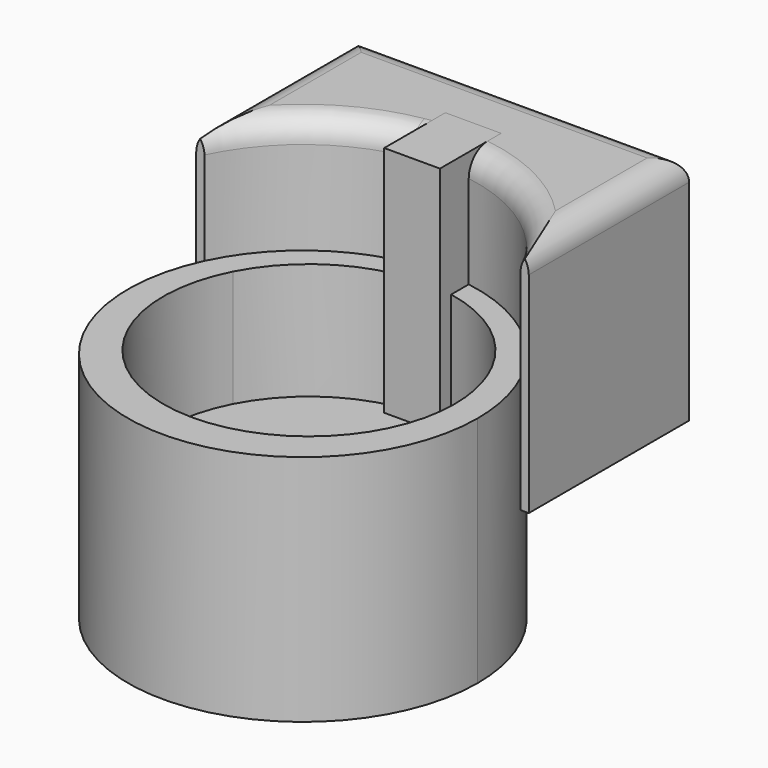
from build123d import *

# Parameters (mm, degrees)
F1_DEPTH    = 50.8
F2_DEPTH    = 25.4
F3_DEPTH    = 25.4
F4_T1_DEPTH = 97.86927917
F4_T3_DEPTH = 69.072270802
F4_T6_ANGLE = 93.763795783
F4_T8_ANGLE = 93.763795783
F5_DEPTH    = 50.8


# Not quite as in the source:
# - a fillet or chamfer that OpenCascade refuses, or shapes differently, is made with other operations: its cross-section is extruded or revolved along the edge and cut away or added


with BuildPart() as f1:
    # F0 (on Top) → F1 (new body)
    with BuildSketch(Plane.XY):
        with BuildLine():
            ThreePointArc((6.0717510059, 35.9461629091), (22.9027694367, 28.7809581965), (34.4542698124, 14.5969468084))
            Line((34.4542698124, 14.5969468084), (36.234639585, 14.5969468084))
            Line((36.234639585, 14.5969468084), (36.234639585, 58.2692176104))
            Line((36.234639585, 58.2692176104), (-36.234639585, 58.2692176104))
            Line((-36.234639585, 58.2692176104), (-36.234639585, 14.5969468084))
            Line((-36.234639585, 14.5969468084), (-34.4542698124, 14.5969468084))
            ThreePointArc((-34.4542698124, 14.5969468084), (-22.9027694367, 28.7809581965), (-6.0717510059, 35.9461629091))
            Line((-6.0717510059, 35.9461629091), (-6.0717510059, 44.7598363188))
            Line((-6.0717510059, 44.7598363188), (6.0717510059, 44.7598363188))
            Line((6.0717510059, 44.7598363188), (6.0717510059, 35.9461629091))
        make_face()
    extrude(amount=F1_DEPTH)

    # F4: fillet of radius 5.08 on 5 edges, made by hand

    # F4_s2 → F4_t1 (cut)
    with BuildSketch(Plane.YZ.offset(-48.934639585)):
        with BuildLine():
            ThreePointArc((58.2692176104, 45.72), (56.7813200588, 49.3121024484), (53.1892176104, 50.8))
            Line((53.1892176104, 50.8), (58.2692176104, 50.8))
            Line((58.2692176104, 50.8), (58.2692176104, 45.72))
        make_face()
    extrude(amount=F4_T1_DEPTH, mode=Mode.SUBTRACT)

    # F4_s4 → F4_t3 (cut)
    with BuildSketch(Plane.XZ.offset(-70.9692176104)):
        with BuildLine():
            ThreePointArc((36.234639585, 45.72), (34.7467420334, 49.3121024484), (31.154639585, 50.8))
            Line((31.154639585, 50.8), (36.234639585, 50.8))
            Line((36.234639585, 50.8), (36.234639585, 45.72))
        make_face()
        with BuildLine():
            ThreePointArc((-36.234639585, 45.72), (-34.7467420334, 49.3121024484), (-31.154639585, 50.8))
            Line((-31.154639585, 50.8), (-36.234639585, 50.8))
            Line((-36.234639585, 50.8), (-36.234639585, 45.72))
        make_face()
    extrude(amount=F4_T3_DEPTH, mode=Mode.SUBTRACT)

    # F4_s5 → F4_t6 (revolve, cut)
    with BuildSketch(Plane(origin=(-0.2831878776, -0.0495849538, 0), x_dir=(0, 0, 1), z_dir=(-0.9850144718, -0.1724717085, 0))):
        with BuildLine():
            ThreePointArc((45.72, 36.4580618529), (49.3121024484, 37.9459594044), (50.8, 41.5380618529))
            Line((50.8, 41.5380618529), (50.8, 36.4580618529))
            Line((50.8, 36.4580618529), (45.72, 36.4580618529))
        make_face()
    revolve(axis=Axis((0, -1.6669177906, 50.8), (0, 0, -1)), revolution_arc=F4_T6_ANGLE, mode=Mode.SUBTRACT)

    # F4_s7 → F4_t8 (revolve, cut)
    with BuildSketch(Plane(origin=(-0.1780570086, -1.6476759621, 0), x_dir=(0, 0, 1), z_dir=(-0.1074400196, -0.9942115681, 0))):
        with BuildLine():
            ThreePointArc((45.72, 37.9209063199), (49.3121024484, 39.4088038715), (50.8, 43.0009063199))
            Line((50.8, 43.0009063199), (50.8, 37.9209063199))
            Line((50.8, 37.9209063199), (45.72, 37.9209063199))
        make_face()
    revolve(axis=Axis((0, -1.6669177906, 50.8), (0, 0, -1)), revolution_arc=F4_T8_ANGLE, mode=Mode.SUBTRACT)


with BuildPart() as f2:
    # F0 (on Top) → F2 (new body, symmetric)
    with BuildSketch(Plane.XY):
        with BuildLine():
            ThreePointArc((-34.4542698124, 14.5969468084), (-8.3337362614, -38.8443146861), (38.1, -1.6669177906))
            ThreePointArc((38.1, -1.6669177906), (37.1773968955, 6.6668184707), (34.4542698124, 14.5969468084))
            Line((34.4542698124, 14.5969468084), (28.1955961787, 14.5969468084))
            ThreePointArc((28.1955961787, 14.5969468084), (30.8486035233, 7.5117348637), (31.75, 0))
            ThreePointArc((31.75, 0), (-7.5117348637, -30.8486035233), (-28.1955961787, 14.5969468084))
            Line((-28.1955961787, 14.5969468084), (-34.4542698124, 14.5969468084))
        make_face()
        with BuildLine():
            Line((28.1955961787, 14.5969468084), (34.4542698124, 14.5969468084))
            ThreePointArc((34.4542698124, 14.5969468084), (22.9027694367, 28.7809581965), (6.0717510059, 35.9461629091))
            Line((6.0717510059, 35.9461629091), (6.0717510059, 31.1640231633))
            ThreePointArc((6.0717510059, 31.1640231633), (19.0310213994, 25.414222878), (28.1955961787, 14.5969468084))
        make_face()
        with BuildLine():
            ThreePointArc((-6.0717510059, 35.9461629091), (-22.9027694367, 28.7809581965), (-34.4542698124, 14.5969468084))
            Line((-34.4542698124, 14.5969468084), (-28.1955961787, 14.5969468084))
            ThreePointArc((-28.1955961787, 14.5969468084), (-19.0310213994, 25.414222878), (-6.0717510059, 31.1640231633))
            Line((-6.0717510059, 31.1640231633), (-6.0717510059, 35.9461629091))
        make_face()
    extrude(amount=F2_DEPTH, both=True)


with BuildPart() as f3:
    # F0 (on Top) → F3 (new body)
    with BuildSketch(Plane.XY):
        with BuildLine():
            ThreePointArc((31.75, 0), (30.8486035233, 7.5117348637), (28.1955961787, 14.5969468084))
            Line((28.1955961787, 14.5969468084), (-28.1955961787, 14.5969468084))
            ThreePointArc((-28.1955961787, 14.5969468084), (-7.5117348637, -30.8486035233), (31.75, 0))
        make_face()
        with BuildLine():
            Line((-28.1955961787, 14.5969468084), (28.1955961787, 14.5969468084))
            ThreePointArc((28.1955961787, 14.5969468084), (19.0310213994, 25.414222878), (6.0717510059, 31.1640231633))
            Line((6.0717510059, 31.1640231633), (6.0717510059, 28.1063281))
            Line((6.0717510059, 28.1063281), (-6.0717510059, 28.1063281))
            Line((-6.0717510059, 28.1063281), (-6.0717510059, 31.1640231633))
            ThreePointArc((-6.0717510059, 31.1640231633), (-19.0310213994, 25.414222878), (-28.1955961787, 14.5969468084))
        make_face()
    extrude(amount=-F3_DEPTH)


with BuildPart() as f5:
    # F0 (on Top) → F5 (new body)
    with BuildSketch(Plane.XY):
        with BuildLine():
            Line((6.0717510059, 31.1640231633), (6.0717510059, 35.9461629091))
            ThreePointArc((6.0717510059, 35.9461629091), (0, 36.4330822094), (-6.0717510059, 35.9461629091))
            Line((-6.0717510059, 35.9461629091), (-6.0717510059, 31.1640231633))
            ThreePointArc((-6.0717510059, 31.1640231633), (0, 31.75), (6.0717510059, 31.1640231633))
        make_face()
        with BuildLine():
            ThreePointArc((-6.0717510059, 35.9461629091), (0, 36.4330822094), (6.0717510059, 35.9461629091))
            Line((6.0717510059, 35.9461629091), (6.0717510059, 44.7598363188))
            Line((6.0717510059, 44.7598363188), (-6.0717510059, 44.7598363188))
            Line((-6.0717510059, 44.7598363188), (-6.0717510059, 35.9461629091))
        make_face()
        with BuildLine():
            Line((6.0717510059, 28.1063281), (6.0717510059, 31.1640231633))
            ThreePointArc((6.0717510059, 31.1640231633), (0, 31.75), (-6.0717510059, 31.1640231633))
            Line((-6.0717510059, 31.1640231633), (-6.0717510059, 28.1063281))
            Line((-6.0717510059, 28.1063281), (6.0717510059, 28.1063281))
        make_face()
    extrude(amount=F5_DEPTH)


solid = Compound([f1.part, f2.part, f3.part, f5.part])
